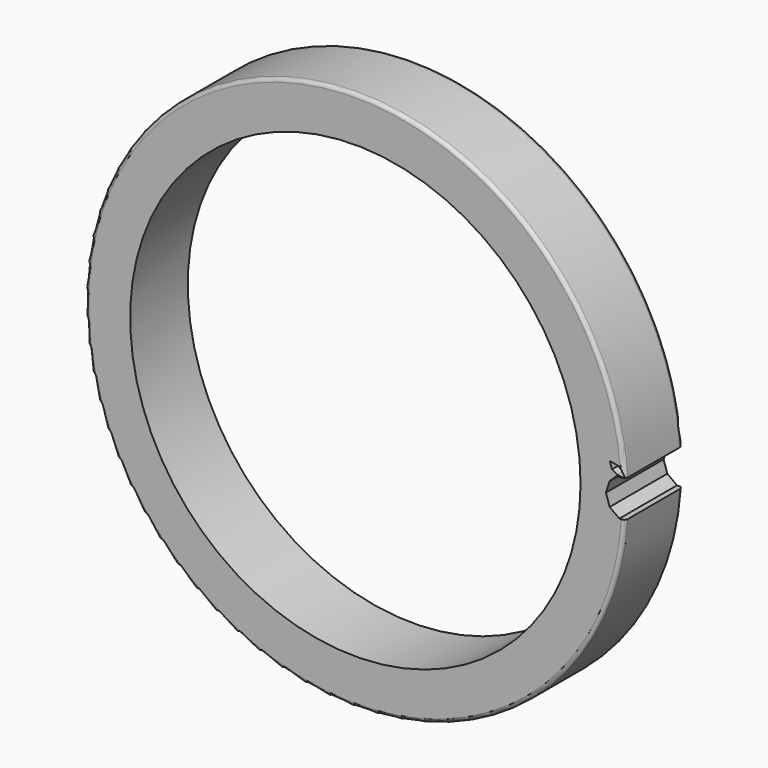
from build123d import *

# Parameters (mm, degrees)
F0_R        = 15
F0_R_2      = 12.5
F2_DEPTH    = 2
F3_DEPTH    = 2
F5_T2_ANGLE = 356.0811167668
F5_T4_ANGLE = 356.0811167668


# Not quite as in the source:
# - a fillet or chamfer that OpenCascade refuses, or shapes differently, is made with other operations: its cross-section is extruded or revolved along the edge and cut away or added


with BuildPart() as f2:
    # F0 (on Front) → F2 (new body, symmetric)
    with BuildSketch(Plane.XZ):
        Circle(F0_R)
        Circle(F0_R_2, mode=Mode.SUBTRACT)
    extrude(amount=F2_DEPTH, both=True)


with BuildPart() as f3:
    # F1 (on Front) → F3 (new body, symmetric)
    with BuildSketch(Plane.XZ):
        Polygon((14.1155660557, -0.6062071938), (14.654473997, -0.9977467319), (15.3206008461, -0.9977467319), (15.8595087875, -0.6062071938), (16.0653533043, 0.0273170867), (15.8595087875, 0.6608413673), (15.4207458886, 1.032837417), (14.98814394, 1.032837417), (14.4956499742, 1.032837417), (14.1155660557, 0.6608413673), (13.9097215389, 0.0273170867), align=None)
    extrude(amount=F3_DEPTH, both=True)


with BuildPart() as f3b:
    # F1 (on Front) → F3, piece 2 (new body, symmetric)
    with BuildSketch(Plane.XZ):
        Polygon((14.5303690806, 1.108682598), (14.9253355339, 1.0592561448), (14.7739350796, 1.3965530088), (14.6046532318, 1.5607766109), (14.1262672842, 1.6433858545), (14.2477648333, 1.2773335911), align=None)
    extrude(amount=F3_DEPTH, both=True)


with BuildPart() as f3c:
    # F1 (on Front) → F3, piece 3 (new body, symmetric)
    with BuildSketch(Plane.XZ):
        Polygon((15.1731697154, 1.4260609763), (14.9909034371, 1.0592561448), (15.3603749383, 1.0987263252), (15.5725924471, 1.2016314485), (15.8138373742, 1.622913168), (15.4283061543, 1.6339400652), align=None)
    extrude(amount=F3_DEPTH, both=True)


with BuildPart() as f2_1:
    add(f2.part)

    # F4: cut F3, F3c, F3b
    add(f3.part, mode=Mode.SUBTRACT)
    add(f3c.part, mode=Mode.SUBTRACT)
    add(f3b.part, mode=Mode.SUBTRACT)

    # F5: fillet of radius 0.2 on 2 edges, made by hand

    # F5_s1 → F5_t2 (revolve, cut)
    with BuildSketch(Plane(origin=(0, 0, 0), x_dir=(0, 1, 0), z_dir=(0.0353637111, 0, -0.9993745084))):
        with BuildLine():
            ThreePointArc((-1.8, 15), (-1.9414213562, 14.9414213562), (-2, 14.8))
            Line((-2, 14.8), (-2, 15))
            Line((-2, 15), (-1.8, 15))
        make_face()
    revolve(axis=Axis((0, -2, 0), (0, -1, 0)), revolution_arc=F5_T2_ANGLE, mode=Mode.SUBTRACT)

    # F5_s3 → F5_t4 (revolve, cut)
    with BuildSketch(Plane(origin=(0, 0, 0), x_dir=(0, 1, 0), z_dir=(0.0353637111, 0, -0.9993745084))):
        with BuildLine():
            ThreePointArc((1.8, 15), (1.9414213562, 14.9414213562), (2, 14.8))
            Line((2, 14.8), (2, 15))
            Line((2, 15), (1.8, 15))
        make_face()
    revolve(axis=Axis((0, 2, 0), (0, -1, 0)), revolution_arc=F5_T4_ANGLE, mode=Mode.SUBTRACT)


solid = f2_1.part
